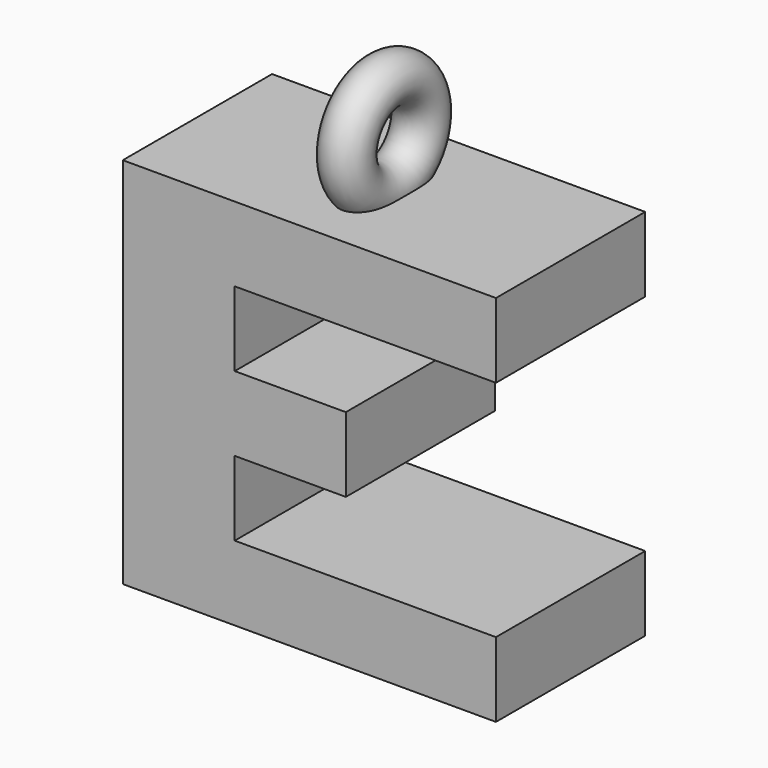
from build123d import *

# Parameters (mm, degrees)
F0_W     = 25.4
F0_H     = 25.4
F1_DEPTH = 12.7
F3_DEPTH = 25.4
F5_R     = 1.5875


# Not quite as in the source:
# - a feature names something its author has since deleted; it is built from what else it names


with BuildPart() as f1:
    # F0 (on Front) → F1 (new body)
    with BuildSketch(Plane.XZ):
        with Locations((12.7, 12.7)):
            Rectangle(F0_W, F0_H)
    extrude(amount=F1_DEPTH)

    # F2 (on face) → F3 (cut)
    with BuildSketch(Plane.XZ.offset(12.7)):
        Polygon((25.4, 5.08), (25.4, 20.32), (7.62, 20.32), (7.62, 15.24), (15.1830166578, 15.24), (15.1830166578, 10.16), (7.62, 10.16), (7.62, 5.08), align=None)
    extrude(amount=-F3_DEPTH, mode=Mode.SUBTRACT)

    # F5 (on offset) → F6 (revolve)
    with BuildSketch(Plane.XZ.offset(6.35)):
        with Locations((12.7, 25.4)):
            Circle(F5_R)
    revolve(axis=Axis((14.955827035, -6.35, 28.575), (1, 0, 0)))


solid = f1.part
